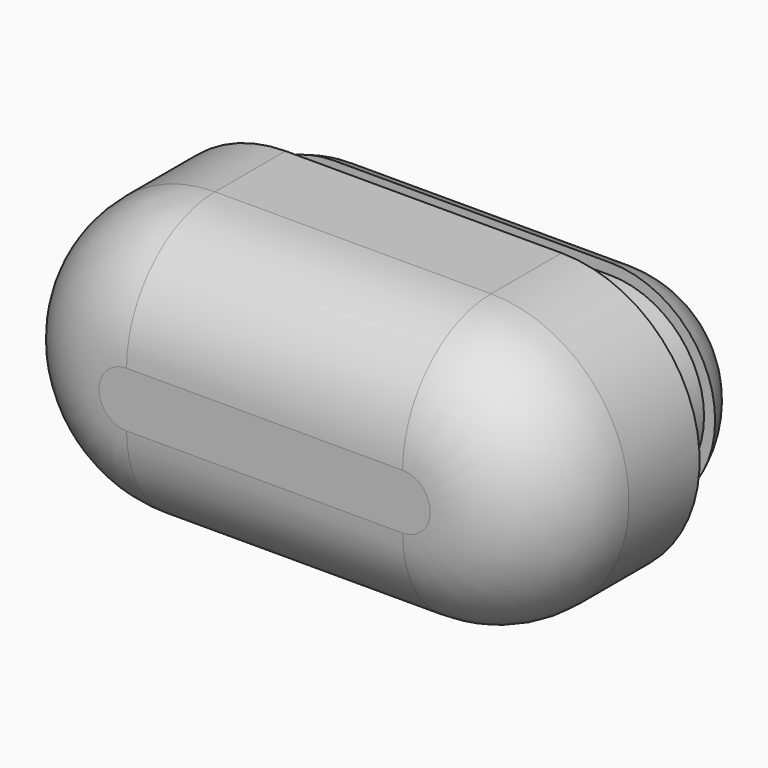
from build123d import *

# Parameters (mm, degrees)
F1_DEPTH    = 9.144
F3_DEPTH    = 2.794
F5_DEPTH    = 3.2766
F6_T1_DEPTH = 12.7
F6_T4_ANGLE = 180
F6_T6_ANGLE = 180
F7_R        = 5.08


# Not quite as in the source:
# - a fillet or chamfer that OpenCascade refuses, or shapes differently, is made with other operations: its cross-section is extruded or revolved along the edge and cut away or added


with BuildPart() as f1:
    # F0 (on Front) → F1 (new body)
    with BuildSketch(Plane.XZ):
        with BuildLine():
            Line((12.7, 12.7), (0, 12.7))
            ThreePointArc((0, 12.7), (-6.35, 6.35), (0, 0))
            Line((0, 0), (12.7, 0))
            ThreePointArc((12.7, 0), (19.05, 6.35), (12.7, 12.7))
        make_face()
    extrude(amount=F1_DEPTH)

    # F2 (on face) → F3 (join)
    with BuildSketch(Plane(origin=(0, 0, 0), x_dir=(-1, 0, 0), z_dir=(0, 1, 0))):
        with BuildLine():
            ThreePointArc((0, 2.032), (4.318, 6.35), (0, 10.668))
            Line((0, 10.668), (-12.7, 10.668))
            ThreePointArc((-12.7, 10.668), (-17.018, 6.35), (-12.7, 2.032))
            Line((-12.7, 2.032), (0, 2.032))
        make_face()
    extrude(amount=F3_DEPTH)

    # F4 (on face) → F5 (join)
    with BuildSketch(Plane(origin=(0, 2.794, 0), x_dir=(-1, 0, 0), z_dir=(0, 1, 0))):
        with BuildLine():
            Line((-12.7, 1.524), (0, 1.524))
            ThreePointArc((0, 1.524), (4.826, 6.35), (0, 11.176))
            Line((0, 11.176), (-12.7, 11.176))
            ThreePointArc((-12.7, 11.176), (-17.526, 6.35), (-12.7, 1.524))
        make_face()
    extrude(amount=F5_DEPTH)

    # F6: fillet of radius 5.08 on 4 edges, made by hand

    # F6_s2 → F6_t1 (cut)
    with BuildSketch(Plane.YZ):
        with BuildLine():
            ThreePointArc((2.794, 11.176), (5.1719677188, 9.3117646326), (6.0706, 6.4268791929))
            Line((6.0706, 6.4268791929), (6.0706, 11.176))
            Line((6.0706, 11.176), (2.794, 11.176))
        make_face()
        with BuildLine():
            ThreePointArc((2.794, 1.524), (5.1719677188, 3.3882353674), (6.0706, 6.2731208071))
            Line((6.0706, 6.2731208071), (6.0706, 1.524))
            Line((6.0706, 1.524), (2.794, 1.524))
        make_face()
    extrude(amount=F6_T1_DEPTH, mode=Mode.SUBTRACT)

    # F6_s3 → F6_t4 (revolve, cut)
    with BuildSketch(Plane.YZ.offset(12.7)):
        with BuildLine():
            ThreePointArc((2.794, 11.176), (5.1719677188, 9.3117646326), (6.0706, 6.4268791929))
            Line((6.0706, 6.4268791929), (6.0706, 11.176))
            Line((6.0706, 11.176), (2.794, 11.176))
        make_face()
    revolve(axis=Axis((12.7, 6.0706, 6.35), (0, 1, 0)), revolution_arc=F6_T4_ANGLE, mode=Mode.SUBTRACT)

    # F6_s5 → F6_t6 (revolve, cut)
    with BuildSketch(Plane.YZ):
        with BuildLine():
            ThreePointArc((6.0706, 6.2731208071), (5.1719677188, 3.3882353674), (2.794, 1.524))
            Line((2.794, 1.524), (6.0706, 1.524))
            Line((6.0706, 1.524), (6.0706, 6.2731208071))
        make_face()
    revolve(axis=Axis((0, 6.0706, 6.35), (0, 1, 0)), revolution_arc=F6_T6_ANGLE, mode=Mode.SUBTRACT)

    # F7
    f7_edges = [f1.edges().sort_by_distance(p)[0] for p in [
        (6.35, -9.144, 12.7),
        (19.05, -9.144, 6.35),
        (6.35, -9.144, 0),
        (-6.35, -9.144, 6.35),
    ]]
    fillet(f7_edges, radius=F7_R)


solid = f1.part
